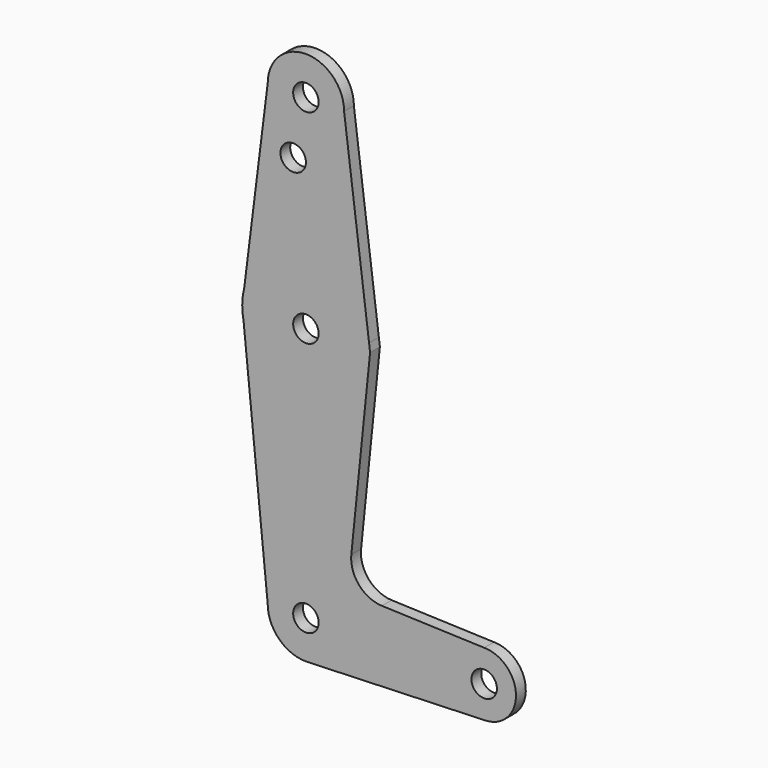
from build123d import *

# Parameters (mm, degrees)
F0_R     = 3.175
F1_DEPTH = 3.048


with BuildPart() as f1:
    # F0 (on Front) → F1 (new body)
    with BuildSketch(Plane.XZ):
        with BuildLine():
            ThreePointArc((0.6773435479, -9.500885786), (6.9705567315, -6.4912990883), (9.525, 0))
            ThreePointArc((9.525, 0), (0, 9.525), (-9.525, 0))
            ThreePointArc((-9.525, 0), (-6.7351920908, -6.7351920908), (0, -9.525))
            Line((0, -9.525), (0.6773435479, -9.500885786))
        make_face()
        Circle(F0_R, mode=Mode.SUBTRACT)
        with BuildLine():
            ThreePointArc((-9.525, 0), (0, 9.525), (9.525, 0))
            ThreePointArc((9.525, 0), (6.9705567315, -6.4912990883), (0.6773435479, -9.500885786))
            Line((0.6773435479, -9.500885786), (44.7324052746, -7.9324746146))
            ThreePointArc((44.7324052746, -7.9324746146), (36.5137564458, -0.1412249921), (44.45, 7.9375))
            Line((44.45, 7.9375), (18.946067877, 8.8483547187))
            ThreePointArc((18.946067877, 8.8483547187), (13.2356131344, 11.5709293815), (11.3206795075, 17.6004181962))
            Line((11.3206795075, 17.6004181962), (16.0035761028, 63.5))
            Line((16.0035761028, 63.5), (15.7474569259, 65.508289164))
            ThreePointArc((15.7474569259, 65.508289164), (15.8430821449, 64.5061675559), (15.875, 63.5))
            ThreePointArc((15.875, 63.5), (1.5796215395, 47.7037846054), (-15.5606435644, 60.3564356436))
            Line((-15.5606435644, 60.3564356436), (-9.525, 0))
        make_face()
        with BuildLine():
            ThreePointArc((0, -9.525), (0.3388863295, -9.5189695375), (0.6773435479, -9.500885786))
            Line((0.6773435479, -9.500885786), (0, -9.525))
        make_face()
        with BuildLine():
            Line((-15.875, 63.5), (-15.5606435644, 60.3564356436))
            ThreePointArc((-15.5606435644, 60.3564356436), (1.5796215395, 47.7037846054), (15.875, 63.5))
            ThreePointArc((15.875, 63.5), (15.8430821449, 64.5061675559), (15.7474569259, 65.508289164))
            ThreePointArc((15.7474569259, 65.508289164), (0.966694683, 79.3455396371), (-15.3865384615, 67.4076923077))
            Line((-15.3865384615, 67.4076923077), (-15.875, 63.5))
        make_face()
        with Locations((0, 63.5)):
            Circle(F0_R, mode=Mode.SUBTRACT)
        with BuildLine():
            ThreePointArc((-15.875, 63.5), (-15.7962153946, 61.9203784605), (-15.5606435644, 60.3564356436))
            Line((-15.5606435644, 60.3564356436), (-15.875, 63.5))
        make_face()
        with BuildLine():
            ThreePointArc((44.45, 7.9375), (36.5137564458, -0.1412249921), (44.7324052746, -7.9324746146))
            ThreePointArc((44.7324052746, -7.9324746146), (50.1616327839, -5.5119104847), (52.3875, 0))
            ThreePointArc((52.3875, 0), (50.0626600757, 5.6126600757), (44.45, 7.9375))
        make_face()
        with Locations((44.45, 0)):
            Circle(F0_R, mode=Mode.SUBTRACT)
        with BuildLine():
            ThreePointArc((-15.3865384615, 67.4076923077), (-15.7524112928, 65.4690514116), (-15.875, 63.5))
            Line((-15.875, 63.5), (-15.3865384615, 67.4076923077))
        make_face()
        with BuildLine():
            Line((-9.525, 114.3), (-15.3865384615, 67.4076923077))
            ThreePointArc((-15.3865384615, 67.4076923077), (0.966694683, 79.3455396371), (15.7474569259, 65.508289164))
            Line((15.7474569259, 65.508289164), (9.525, 114.3))
            ThreePointArc((9.525, 114.3), (0, 104.775), (-9.525, 114.3))
        make_face()
        with Locations((-3.175, 100.0252)):
            Circle(F0_R, mode=Mode.SUBTRACT)
        with BuildLine():
            ThreePointArc((9.525, 114.3), (0, 123.825), (-9.525, 114.3))
            ThreePointArc((-9.525, 114.3), (0, 104.775), (9.525, 114.3))
        make_face()
        with Locations((0, 114.3)):
            Circle(F0_R, mode=Mode.SUBTRACT)
    extrude(amount=F1_DEPTH)


solid = f1.part
